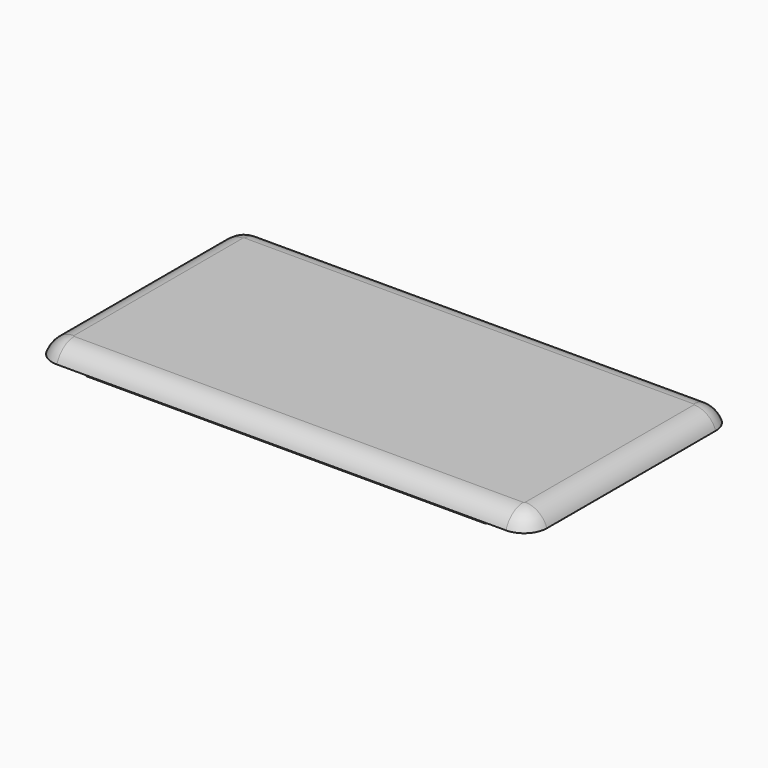
from build123d import *

# Parameters (mm, degrees)
F1_DEPTH     = 3.5
F5_D         = 4.473
F5_DEPTH     = 0.8
F5_TIP       = 1.3438247745
F6_T1_DEPTH  = 99
F6_T3_DEPTH  = 46.5
F6_T6_ANGLE  = 90
F6_T8_ANGLE  = 90
F6_T10_ANGLE = 90
F6_T12_ANGLE = 90
F8_W         = 0.5
F8_H         = 37.5
F8_W_2       = 88
F8_H_2       = 0.5
F9_DEPTH     = 1


# Not quite as in the source:
# - a fillet or chamfer that OpenCascade refuses, or shapes differently, is made with other operations: its cross-section is extruded or revolved along the edge and cut away or added


with BuildPart() as f1:
    # F0 (on Top) → F1 (new body)
    with BuildSketch(Plane.XY):
        with BuildLine():
            Line((-49.5, -28.25), (49.5, -28.25))
            ThreePointArc((49.5, -28.25), (53.0355339059, -26.7855339059), (54.5, -23.25))
            Line((54.5, -23.25), (54.5, 23.25))
            ThreePointArc((54.5, 23.25), (53.0355339059, 26.7855339059), (49.5, 28.25))
            Line((49.5, 28.25), (-49.5, 28.25))
            ThreePointArc((-49.5, 28.25), (-53.0355339059, 26.7855339059), (-54.5, 23.25))
            Line((-54.5, 23.25), (-54.5, -23.25))
            ThreePointArc((-54.5, -23.25), (-53.0355339059, -26.7855339059), (-49.5, -28.25))
        make_face()
    extrude(amount=F1_DEPTH)

    # F5
    with Locations(Plane(origin=(0, 0, 0), x_dir=(1, 0, 0), z_dir=(0, 0, -1))):
        with Locations((-50.2406740561, -23.9985361695), (-50.2495961264, 24.0030474961), (50.2488752827, 23.995583877), (50.2413948998, -24.0000952035)):
            Hole(F5_D / 2, depth=F5_DEPTH)
            with Locations((0, 0, -(F5_DEPTH + F5_TIP / 2))):  # 118° drill point
                Cone(0, F5_D / 2, F5_TIP, mode=Mode.SUBTRACT)

    # F6: fillet of radius 5 on 1 edges, made by hand

    # F6_s2 → F6_t1 (cut)
    with BuildSketch(Plane.YZ.offset(-49.5)):
        with BuildLine():
            ThreePointArc((-28.25, 0), (-26.4383438845, 2.5311288741), (-23.4803039929, 3.5))
            Line((-23.4803039929, 3.5), (-28.25, 3.5))
            Line((-28.25, 3.5), (-28.25, 0))
        make_face()
        with BuildLine():
            ThreePointArc((23.4803039929, 3.5), (26.4383438845, 2.5311288741), (28.25, 0))
            Line((28.25, 0), (28.25, 3.5))
            Line((28.25, 3.5), (23.4803039929, 3.5))
        make_face()
    extrude(amount=F6_T1_DEPTH, mode=Mode.SUBTRACT)

    # F6_s4 → F6_t3 (cut)
    with BuildSketch(Plane.XZ.offset(-23.25)):
        with BuildLine():
            ThreePointArc((49.7303039929, 3.5), (52.6883438845, 2.5311288741), (54.5, 0))
            Line((54.5, 0), (54.5, 3.5))
            Line((54.5, 3.5), (49.7303039929, 3.5))
        make_face()
        with BuildLine():
            ThreePointArc((-49.7303039929, 3.5), (-52.6883438845, 2.5311288741), (-54.5, 0))
            Line((-54.5, 0), (-54.5, 3.5))
            Line((-54.5, 3.5), (-49.7303039929, 3.5))
        make_face()
    extrude(amount=F6_T3_DEPTH, mode=Mode.SUBTRACT)

    # F6_s5 → F6_t6 (revolve, cut)
    with BuildSketch(Plane.XZ.offset(23.25)):
        with BuildLine():
            ThreePointArc((-54.5, 0), (-52.6883438845, 2.5311288741), (-49.7303039929, 3.5))
            Line((-49.7303039929, 3.5), (-54.5, 3.5))
            Line((-54.5, 3.5), (-54.5, 0))
        make_face()
    revolve(axis=Axis((-49.5, -23.25, 3.5), (0, 0, 1)), revolution_arc=F6_T6_ANGLE, mode=Mode.SUBTRACT)

    # F6_s7 → F6_t8 (revolve, cut)
    with BuildSketch(Plane.YZ.offset(49.5)):
        with BuildLine():
            ThreePointArc((-28.25, 0), (-26.4383438845, 2.5311288741), (-23.4803039929, 3.5))
            Line((-23.4803039929, 3.5), (-28.25, 3.5))
            Line((-28.25, 3.5), (-28.25, 0))
        make_face()
    revolve(axis=Axis((49.5, -23.25, 3.5), (0, 0, 1)), revolution_arc=F6_T8_ANGLE, mode=Mode.SUBTRACT)

    # F6_s9 → F6_t10 (revolve, cut)
    with BuildSketch(Plane.XZ.offset(-23.25)):
        with BuildLine():
            ThreePointArc((49.7303039929, 3.5), (52.6883438845, 2.5311288741), (54.5, 0))
            Line((54.5, 0), (54.5, 3.5))
            Line((54.5, 3.5), (49.7303039929, 3.5))
        make_face()
    revolve(axis=Axis((49.5, 23.25, 3.5), (0, 0, 1)), revolution_arc=F6_T10_ANGLE, mode=Mode.SUBTRACT)

    # F6_s11 → F6_t12 (revolve, cut)
    with BuildSketch(Plane.YZ.offset(-49.5)):
        with BuildLine():
            ThreePointArc((23.4803039929, 3.5), (26.4383438845, 2.5311288741), (28.25, 0))
            Line((28.25, 0), (28.25, 3.5))
            Line((28.25, 3.5), (23.4803039929, 3.5))
        make_face()
    revolve(axis=Axis((-49.5, 23.25, 3.5), (0, 0, 1)), revolution_arc=F6_T12_ANGLE, mode=Mode.SUBTRACT)

    # F8 (on Top) → F9 (join)
    with BuildSketch(Plane.XY):
        with Locations((-53.0630070642, -0.0139670707)):
            Rectangle(F8_W, F8_H)
        with Locations((-0.0016481951, -26.7570052035)):
            Rectangle(F8_W_2, F8_H_2)
        with Locations((53.0663034543, -0.0139678158)):
            Rectangle(F8_W, F8_H)
        with Locations((-0.0016481951, 26.78494009)):
            Rectangle(F8_W_2, F8_H_2)
    extrude(amount=-F9_DEPTH)


solid = f1.part
